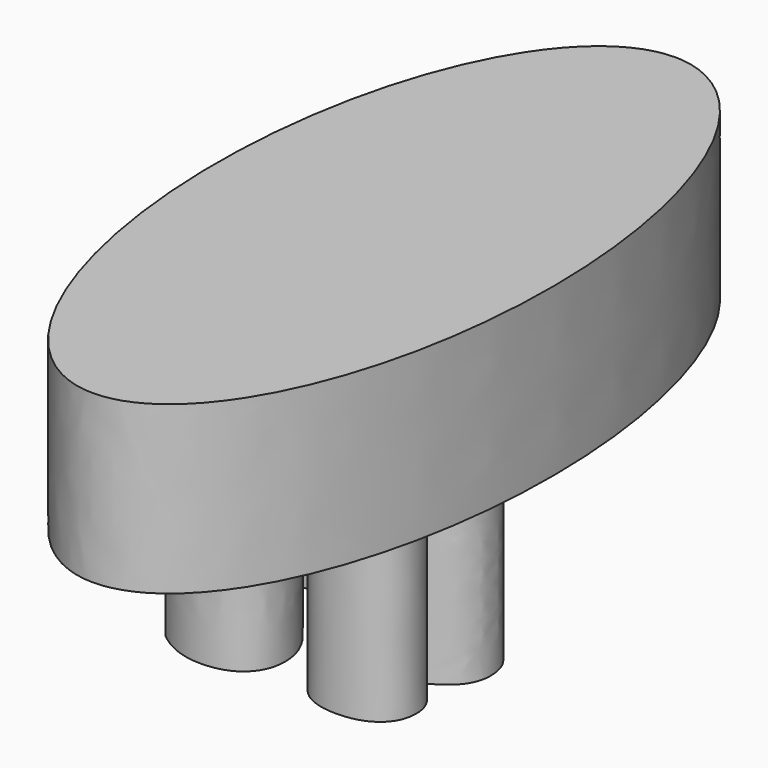
from build123d import *

# Parameters (mm, degrees)
F1_DEPTH     = 30.226
F3_TEXT_SIZE = 42.0930954868
F4_DEPTH     = 33.528


# Not quite as in the source:
# - Text() gives the source's letters only with a copy of the font that has no kerning and outlines rounded to 1/6400 em; it was checked with that copy


with BuildPart() as f1:
    # F0 (on Top) → F1 (new body)
    with BuildSketch(Plane.XY):
        with BuildLine():
            add(Edge.make_bspline(
                [(0, 65.9713447094), (-52.733007108, 65.9713447094), (-26.366503554, -32.9856723547), (0, -131.9426894188), (26.366503554, -32.9856723547), (52.733007108, 65.9713447094), (0, 65.9713447094)],
                knots=[0, 0, 0, 2.0943951024, 2.0943951024, 4.1887902048, 4.1887902048, 6.2831853072, 6.2831853072, 6.2831853072], degree=2, weights=[1, 0.5, 1, 0.5, 1, 0.5, 1]))
        make_face()
    extrude(amount=F1_DEPTH)

    # F3 (on face) → F4 (join)
    with BuildSketch(Plane(origin=(0, 0, 0), x_dir=(1, 0, 0), z_dir=(0, 0, -1))):
        with Locations((-24.3416478745, -4.9070287505)):
            Text('28', F3_TEXT_SIZE, font='Open Sans', text_align=(TextAlign.LEFT, TextAlign.BOTTOM))
    extrude(amount=F4_DEPTH)


solid = f1.part
